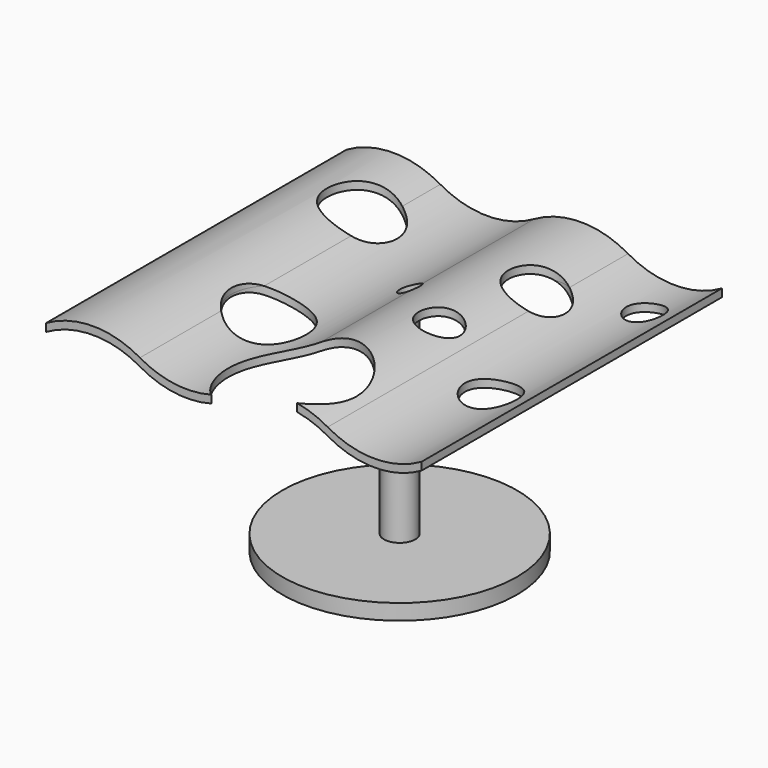
from build123d import *

# Parameters (mm, degrees)
F1_DEPTH = 609.6
F2_R     = 114.3
F2_R_2   = 92.0904361078
F2_R_3   = 121.8366951499
F2_R_4   = 32.9073825218
F2_R_5   = 84.4397606998
F2_R_6   = 59.4014676345
F2_R_7   = 67.0056628832
F2_R_8   = 208.6499704461
F3_DEPTH = 127
F4_R     = 50.8
F5_DEPTH = 635
F6_R     = 381
F6_R_2   = 50.8
F7_DEPTH = 50.8


with BuildPart() as f1:
    # F0 (on Front) → F1 (new body, symmetric)
    with BuildSketch(Plane.XZ):
        with BuildLine():
            Line((-355.6, -25.4), (-355.6, 0))
            ThreePointArc((-355.6, 0), (-508, 40.8354569265), (-660.4, 0))
            Line((-660.4, 0), (-660.4, -25.4))
            ThreePointArc((-660.4, -25.4), (-508, 15.4354569265), (-355.6, -25.4))
        make_face()
        with BuildLine():
            ThreePointArc((-50.8, 0), (-203.2, -40.8354569265), (-355.6, 0))
            Line((-355.6, 0), (-355.6, -25.4))
            ThreePointArc((-355.6, -25.4), (-203.2, -66.2354569265), (-50.8, -25.4))
            Line((-50.8, -25.4), (-50.8, 0))
        make_face()
        with BuildLine():
            ThreePointArc((254, 0), (101.6, 40.8354569265), (-50.8, 0))
            Line((-50.8, 0), (-50.8, -25.4))
            ThreePointArc((-50.8, -25.4), (101.6, 15.4354569265), (254, -25.4))
            Line((254, -25.4), (254, 0))
        make_face()
        with BuildLine():
            ThreePointArc((558.8, 0), (406.4, -40.8354569265), (254, 0))
            Line((254, 0), (254, -25.4))
            ThreePointArc((254, -25.4), (406.4, -66.2354569265), (558.8, -25.4))
            Line((558.8, -25.4), (558.8, 0))
        make_face()
    extrude(amount=F1_DEPTH, both=True)

    # F2 (on Top) → F3 (cut, symmetric)
    with BuildSketch(Plane.XY):
        with Locations((-403.1560122967, 351.4335751534)):
            Circle(F2_R)
        with Locations((214.2508625984, 288.6464297771)):
            Circle(F2_R_2)
        with Locations((-270.6053853035, -192.7216351032)):
            Circle(F2_R_3)
        with Locations((-71.7794522643, 131.6785812378)):
            Circle(F2_R_4)
        with Locations((420.0531244278, -154.3517261744)):
            Circle(F2_R_5)
        with Locations((444.470345974, 438.6379420757)):
            Circle(F2_R_6)
        with Locations((154.9518704414, -32.2656147182)):
            Circle(F2_R_7)
        with Locations((15.4249072075, -454.334706068)):
            Circle(F2_R_8)
    extrude(amount=F3_DEPTH, both=True, mode=Mode.SUBTRACT)

    # F4 (on Top) → F5 (join)
    with BuildSketch(Plane.XY):
        Circle(F4_R)
    extrude(amount=-F5_DEPTH)

    # F6 (on face) → F7 (join)
    with BuildSketch(Plane(origin=(0, 0, -635), x_dir=(1, 0, 0), z_dir=(0, 0, -1))):
        Circle(F6_R)
        Circle(F6_R_2, mode=Mode.SUBTRACT)
        Circle(F6_R_2)
    extrude(amount=F7_DEPTH)


solid = f1.part
